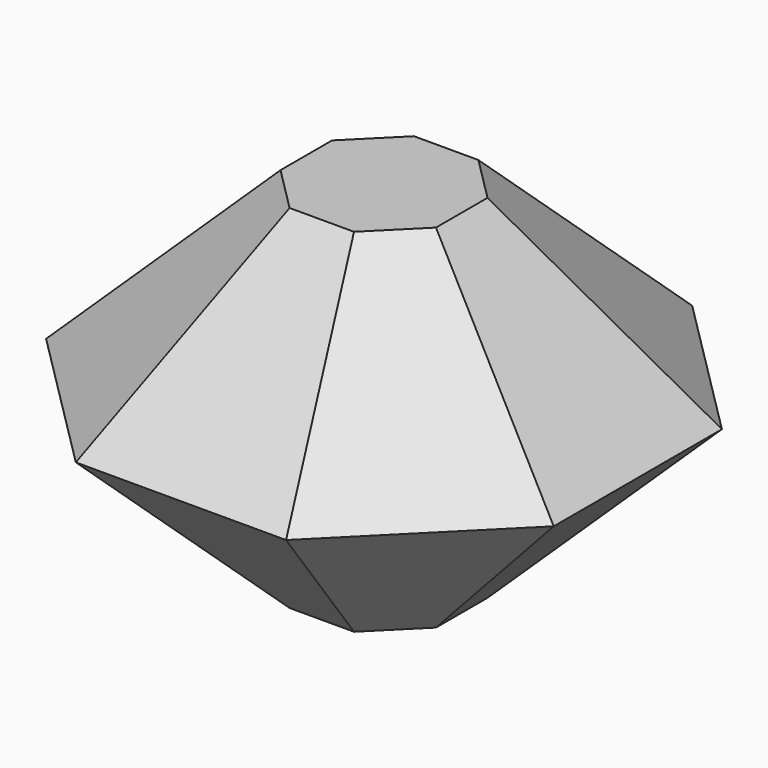
from build123d import *

# Parameters (mm, degrees)
F1_DEPTH = 20
F2_SIZE  = 9.99999


# Not quite as in the source:
# - a fillet or chamfer is up to 0.001 mm smaller than in the source, because OpenCascade refuses the exact size


with BuildPart() as f1:
    # F0 (on Top) → F1 (new body)
    with BuildSketch(Plane.XY):
        Polygon((-5.9708582602, -14.4149269909), (5.9708582602, -14.4149269909), (11.5348123973, -8.8509728538), (14.4149269909, -3.8624680462), (14.4149269909, 3.8624680462), (11.5348123973, 8.8509728538), (5.9708582602, 14.4149269909), (-5.9708582602, 14.4149269909), (-11.5348123973, 8.8509728538), (-14.4149269909, 3.8624680462), (-14.4149269909, -3.8624680462), (-11.5348123973, -8.8509728538), align=None)
        Polygon((-14.4149269909, -5.9708582602), (-11.5348123973, -8.8509728538), (-14.4149269909, -3.8624680462), align=None)
        Polygon((-14.4149269909, 5.9708582602), (-14.4149269909, 3.8624680462), (-11.5348123973, 8.8509728538), align=None)
        Polygon((14.4149269909, -3.8624680462), (11.5348123973, -8.8509728538), (14.4149269909, -5.9708582602), align=None)
        Polygon((11.5348123973, 8.8509728538), (14.4149269909, 3.8624680462), (14.4149269909, 5.9708582602), align=None)
    extrude(amount=F1_DEPTH)

    # F2 (size 10 in the source; OpenCascade refuses exactly that, so slightly less here)
    f2_edges = [f1.edges().sort_by_distance(p)[0] for p in [
        (0, 14.414927, 20),
        (-10.192893, 10.192893, 20),
        (-14.414927, 0, 20),
        (-10.192893, -10.192893, 20),
        (0, -14.414927, 20),
        (10.192893, -10.192893, 20),
        (14.414927, 0, 20),
        (10.192893, 10.192893, 20),
        (0, 14.414927, 0),
        (-10.192893, 10.192893, 0),
        (-14.414927, 0, 0),
        (-10.192893, -10.192893, 0),
        (0, -14.414927, 0),
        (10.192893, -10.192893, 0),
        (14.414927, 0, 0),
        (10.192893, 10.192893, 0),
    ]]
    chamfer(f2_edges, length=F2_SIZE)


solid = f1.part
